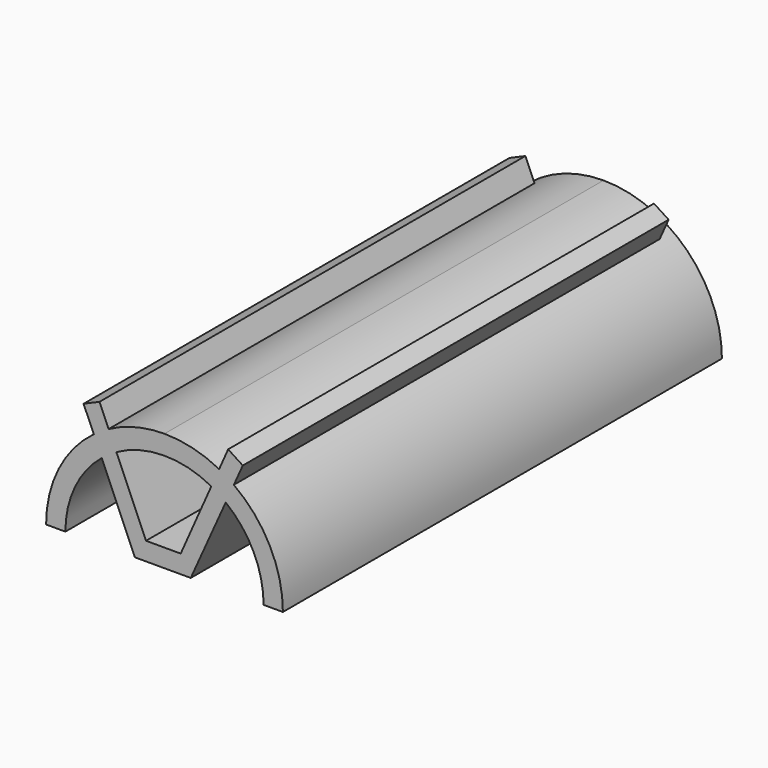
from build123d import *

# Parameters (mm, degrees)
F1_DEPTH = 177.8
F3_DEPTH = 172.466


# Not quite as in the source:
# - a feature names something its author has since deleted; it is built from what else it names


with BuildPart() as f1:
    # F0 (on Front) → F1 (new body)
    with BuildSketch(Plane.XZ):
        with BuildLine():
            ThreePointArc((-32.1100279689, 0), (-22.7052185209, 22.7052185209), (0, 32.1100279689))
            ThreePointArc((0, 32.1100279689), (22.7052185209, 22.7052185209), (32.1100279689, 0))
            Line((32.1100279689, 0), (38.3662581444, 0))
            ThreePointArc((38.3662581444, 0), (27.1290413026, 27.1290413026), (0, 38.3662581444))
            ThreePointArc((0, 38.3662581444), (-27.1290413026, 27.1290413026), (-38.3662581444, 0))
            Line((-38.3662581444, 0), (-32.1100279689, 0))
        make_face()
    extrude(amount=F1_DEPTH)

    # F2 (on face) → F3 (join)
    with BuildSketch(Plane.XZ.offset(177.8)):
        Polygon((-26.2182112783, 38.40040043), (-9.5876645925, 0), (0, 0), (8.5017651877, 0), (25.3681559116, 37.5649854541), (20.6263340544, 40.6422178311), (5.2554043941, 5.8927594628), (-5.9924047246, 5.8927594628), (-21.0417917943, 40.6422178311), align=None)
    extrude(amount=-F3_DEPTH)


solid = f1.part
